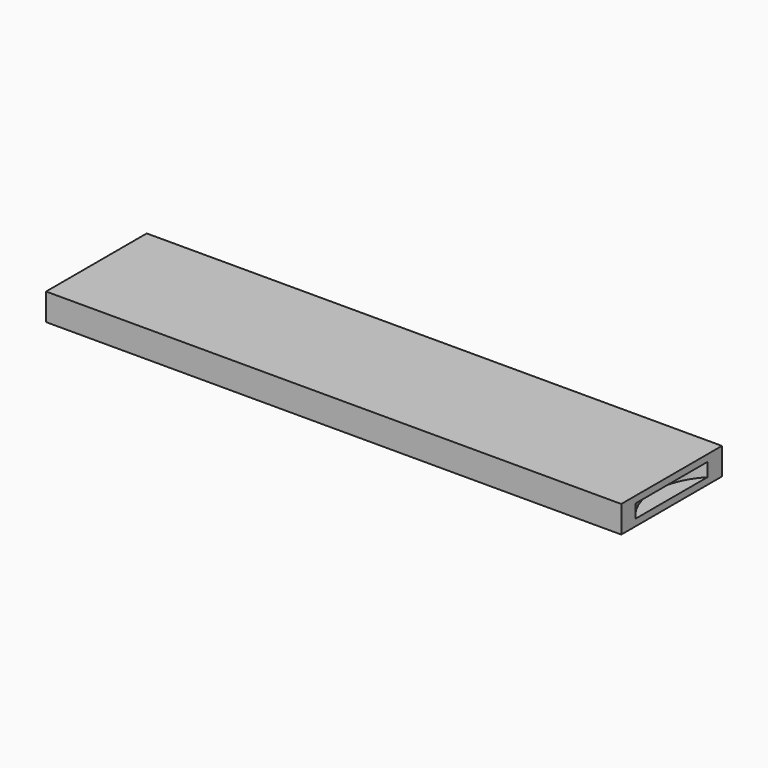
from build123d import *

# Parameters (mm, degrees)
F0_W          = 88.9
F0_H          = 19.05
F1_DEPTH      = 406.4
F3_DEPTH      = 4.7625
F3_DEPTH_BACK = 4.7625


# Not quite as in the source:
# - a pattern or mirror of a feature is missing from the dataset's text; its kind, count and spacing are read off the source's solid


with BuildPart() as f1:
    # F0 (on Right) → F1 (new body)
    with BuildSketch(Plane.YZ):
        Rectangle(F0_W, F0_H)
    extrude(amount=F1_DEPTH)

    # F2 (on Top) → F3 (cut, two sides)
    with BuildSketch(Plane.XY) as f3_sk:
        with BuildLine():
            Line((0, 31.75), (0, -31.75))
            ThreePointArc((0, -31.75), (12.7, 0), (0, 31.75))
        make_face()
    f3 = extrude(amount=F3_DEPTH, mode=Mode.SUBTRACT) + extrude(f3_sk.sketch, amount=-F3_DEPTH_BACK, mode=Mode.SUBTRACT)

    # F3_copies: F3 across plane
    add(f3.mirror(Plane(origin=(203.2, 0, 0), x_dir=(0, 0, 1), z_dir=(1, 0, 0))), mode=Mode.SUBTRACT)


solid = f1.part
